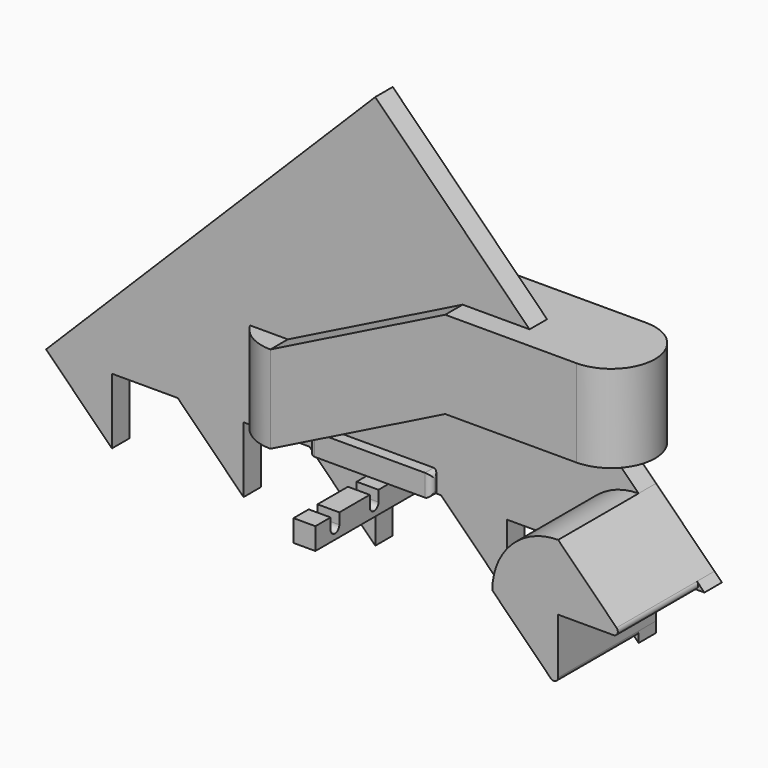
from build123d import *

# Parameters (mm, degrees)
F0_W          = 101.6
F0_H          = 50.8
F0_W_2        = 50.8
F0_H_2        = 101.6
F1_DEPTH      = 50.8
F2_ANGLE_BACK = 90
F2_ANGLE      = 180
F3_DEPTH      = 2.286
F0_W_3        = 43.6525400519
F4_ANGLE_BACK = 90
F4_ANGLE      = 180
F5_W          = 22.098
F5_H          = 6.35
F6_DEPTH      = 25.4
F7_W          = 57.8641055384
F7_H          = 12.7
F7_W_2        = 12.7
F7_H_2        = 49.9071290871
F8_DEPTH      = 25.4
F9_R          = 6.34999
F11_DEPTH     = 25.4
F12_DEPTH     = 142.24
F13_R         = 5.08


# Not quite as in the source:
# - a fillet or chamfer is up to 0.001 mm smaller than in the source, because OpenCascade refuses the exact size


with BuildPart() as f1:
    # F0 (on Front) → F1 (new body, symmetric)
    with BuildSketch(Plane.XZ):
        Polygon((101.6, 203.2), (0, 152.4), (101.6, 152.4), align=None)
        with Locations((50.8, 127)):
            Rectangle(F0_W, F0_H)
        Polygon((0, 152.4), (-101.6, 101.6), (0, 101.6), align=None)
        with Locations((-50.8, 76.2)):
            Rectangle(F0_W, F0_H)
        Polygon((0, 101.6), (0, 50.8), (101.6, 101.6), align=None)
        Polygon((-101.6, 50.8), (-101.6, 0), (0, 50.8), align=None)
        Polygon((101.6, 152.4), (101.6, 101.6), (152.4, 101.6), (152.4, 203.2), (101.6, 203.2), align=None)
        with Locations((177.8, 152.4)):
            Rectangle(F0_W_2, F0_H_2)
        with Locations((228.6, 152.4)):
            Rectangle(F0_W_2, F0_H_2)
    extrude(amount=F1_DEPTH, both=True)

    # F0 (on Front) → F2 (revolve)
    with BuildSketch(Plane.XZ, mode=Mode.PRIVATE) as f2_sk:
        with Locations((279.4, 152.4)):
            Rectangle(F0_W_2, F0_H_2)
    revolve(f2_sk.sketch.rotate(Axis((254, 0, 152.4), (0, 0, -1)), -F2_ANGLE_BACK), axis=Axis((254, 0, 152.4), (0, 0, -1)), revolution_arc=F2_ANGLE)

    # F0 (on Front) → F4 (revolve)
    with BuildSketch(Plane.XZ, mode=Mode.PRIVATE) as f4_sk:
        with Locations((-130.573729974, 50.8)):
            Rectangle(F0_W_3, F0_H_2)
        Polygon((-108.7474599481, 0), (-101.6, 0), (-101.6, 50.8), (-101.6, 101.6), (-108.7474599481, 101.6), align=None)
    revolve(f4_sk.sketch.rotate(Axis((-101.6, 0, 50.8), (0, 0, -1)), -F4_ANGLE_BACK), axis=Axis((-101.6, 0, 50.8), (0, 0, -1)), revolution_arc=F4_ANGLE)


with BuildPart() as f3:
    # F0 (on Front) → F3 (new body)
    with BuildSketch(Plane.XZ):
        Polygon((-108.7474599481, 0), (-101.6, 0), (-101.6, 50.8), (-101.6, 101.6), (-108.7474599481, 101.6), align=None)
    extrude(amount=F3_DEPTH)

    # F10 (on Front) → F11 (join)
    with BuildSketch(Plane.XZ):
        Polygon((-344.3030196818, 38.2558910758), (-382.5589107575, 0), (-306.047128606, 0), align=None)
        Polygon((-306.047128606, 0), (-382.5589107575, 0), (-306.047128606, -76.5117821515), align=None)
        Polygon((-344.3030196818, 38.2558910758), (-306.047128606, 0), (-229.5353464545, 0), (-306.047128606, 76.5117821515), align=None)
        with BuildLine():
            ThreePointArc((-229.5353464545, 0), (-251.945128606, 54.102), (-306.047128606, 76.5117821515))
            Line((-306.047128606, 76.5117821515), (-229.5353464545, 0))
        make_face()
        with BuildLine():
            Line((-267.7912375303, 114.7676732273), (-306.047128606, 76.5117821515))
            ThreePointArc((-306.047128606, 76.5117821515), (-251.945128606, 54.102), (-229.5353464545, 0))
            ThreePointArc((-229.5353464545, 0), (-223.7112338288, 29.2797914101), (-207.125564303, 54.102))
            Line((-207.125564303, 54.102), (-267.7912375303, 114.7676732273))
        make_face()
        with BuildLine():
            ThreePointArc((-207.125564303, 54.102), (-223.7112338288, 29.2797914101), (-229.5353464545, 0))
            Line((-229.5353464545, 0), (-153.023564303, 0))
            Line((-153.023564303, 0), (-207.125564303, 54.102))
        make_face()
        Polygon((-153.023564303, 0), (-229.5353464545, 0), (-153.023564303, -76.5117821515), align=None)
        with BuildLine():
            Line((-229.5353464545, 153.023564303), (-267.7912375303, 114.7676732273))
            Line((-267.7912375303, 114.7676732273), (-207.125564303, 54.102))
            ThreePointArc((-207.125564303, 54.102), (-182.3033557131, 70.6876695257), (-153.023564303, 76.5117821515))
            Line((-153.023564303, 76.5117821515), (-229.5353464545, 153.023564303))
        make_face()
        with BuildLine():
            Line((-207.125564303, 54.102), (-153.023564303, 0))
            Line((-153.023564303, 0), (-76.5117821515, 0))
            Line((-76.5117821515, 0), (-153.023564303, 76.5117821515))
            ThreePointArc((-153.023564303, 76.5117821515), (-182.3033557131, 70.6876695257), (-207.125564303, 54.102))
        make_face()
        with BuildLine():
            Line((-191.2794553788, 191.2794553788), (-229.5353464545, 153.023564303))
            Line((-229.5353464545, 153.023564303), (-153.023564303, 76.5117821515))
            ThreePointArc((-153.023564303, 76.5117821515), (-98.921564303, 54.102), (-76.5117821515, 0))
            ThreePointArc((-76.5117821515, 0), (-70.6876695257, 29.2797914101), (-54.102, 54.102))
            Line((-54.102, 54.102), (-191.2794553788, 191.2794553788))
        make_face()
        Polygon((-38.2558910758, 38.2558910758), (-76.5117821515, 0), (0, 0), align=None)
        Polygon((0, 0), (-76.5117821515, 0), (0, -76.5117821515), align=None)
        with BuildLine():
            ThreePointArc((-54.102, 54.102), (-70.6876695257, 29.2797914101), (-76.5117821515, 0))
            Line((-76.5117821515, 0), (-38.2558910758, 38.2558910758))
            Line((-38.2558910758, 38.2558910758), (-54.102, 54.102))
        make_face()
        with BuildLine():
            Line((-153.023564303, 76.5117821515), (-76.5117821515, 0))
            ThreePointArc((-76.5117821515, 0), (-98.921564303, 54.102), (-153.023564303, 76.5117821515))
        make_face()
        with BuildLine():
            Line((-153.023564303, 229.5353464545), (-191.2794553788, 191.2794553788))
            Line((-191.2794553788, 191.2794553788), (-54.102, 54.102))
            ThreePointArc((-54.102, 54.102), (-29.2797914101, 70.6876695257), (0, 76.5117821515))
            Line((0, 76.5117821515), (-153.023564303, 229.5353464545))
        make_face()
        Polygon((-38.2558910758, 38.2558910758), (0, 0), (76.5117821515, 0), (0, 76.5117821515), align=None)
        with BuildLine():
            Line((-54.102, 54.102), (-38.2558910758, 38.2558910758))
            Line((-38.2558910758, 38.2558910758), (0, 76.5117821515))
            ThreePointArc((0, 76.5117821515), (-29.2797914101, 70.6876695257), (-54.102, 54.102))
        make_face()
        Polygon((-114.7676732273, 267.7912375303), (-153.023564303, 229.5353464545), (0, 76.5117821515), (38.2558910758, 114.7676732273), align=None)
        Polygon((114.7676732273, 38.2558910758), (76.5117821515, 0), (153.023564303, 0), align=None)
        Polygon((153.023564303, 0), (76.5117821515, 0), (153.023564303, -76.5117821515), align=None)
        with BuildLine():
            ThreePointArc((98.921564303, 54.102), (82.3358947773, 29.2797914101), (76.5117821515, 0))
            Line((76.5117821515, 0), (114.7676732273, 38.2558910758))
            Line((114.7676732273, 38.2558910758), (98.921564303, 54.102))
        make_face()
        with BuildLine():
            ThreePointArc((0, 76.5117821515), (54.102, 54.102), (76.5117821515, 0))
            ThreePointArc((76.5117821515, 0), (82.3358947773, 29.2797914101), (98.921564303, 54.102))
            Line((98.921564303, 54.102), (38.2558910758, 114.7676732273))
            Line((38.2558910758, 114.7676732273), (0, 76.5117821515))
        make_face()
        with BuildLine():
            Line((0, 76.5117821515), (76.5117821515, 0))
            ThreePointArc((76.5117821515, 0), (54.102, 54.102), (0, 76.5117821515))
        make_face()
        Polygon((-76.5117821515, 306.047128606), (-114.7676732273, 267.7912375303), (38.2558910758, 114.7676732273), (76.5117821515, 153.023564303), align=None)
        Polygon((114.7676732273, 38.2558910758), (153.023564303, 0), (229.5353464545, 0), (153.023564303, 76.5117821515), align=None)
        with BuildLine():
            Line((98.921564303, 54.102), (114.7676732273, 38.2558910758))
            Line((114.7676732273, 38.2558910758), (153.023564303, 76.5117821515))
            ThreePointArc((153.023564303, 76.5117821515), (123.7437728929, 70.6876695257), (98.921564303, 54.102))
        make_face()
        with BuildLine():
            Line((38.2558910758, 114.7676732273), (98.921564303, 54.102))
            ThreePointArc((98.921564303, 54.102), (123.7437728929, 70.6876695257), (153.023564303, 76.5117821515))
            Line((153.023564303, 76.5117821515), (76.5117821515, 153.023564303))
            Line((76.5117821515, 153.023564303), (38.2558910758, 114.7676732273))
        make_face()
        Polygon((-38.2558910758, 344.3030196818), (-76.5117821515, 306.047128606), (76.5117821515, 153.023564303), (114.7676732273, 191.2794553788), align=None)
        with BuildLine():
            ThreePointArc((251.945128606, 54.102), (235.3594590803, 29.2797914101), (229.5353464545, 0))
            Line((229.5353464545, 0), (306.047128606, 0))
            Line((306.047128606, 0), (251.945128606, 54.102))
        make_face()
        Polygon((306.047128606, 0), (229.5353464545, 0), (306.047128606, -76.5117821515), align=None)
        with BuildLine():
            ThreePointArc((153.023564303, 76.5117821515), (207.125564303, 54.102), (229.5353464545, 0))
            ThreePointArc((229.5353464545, 0), (235.3594590803, 29.2797914101), (251.945128606, 54.102))
            Line((251.945128606, 54.102), (191.2794553788, 114.7676732273))
            Line((191.2794553788, 114.7676732273), (153.023564303, 76.5117821515))
        make_face()
        with BuildLine():
            Line((153.023564303, 76.5117821515), (229.5353464545, 0))
            ThreePointArc((229.5353464545, 0), (207.125564303, 54.102), (153.023564303, 76.5117821515))
        make_face()
        Polygon((153.023564303, 153.023564303), (153.023564303, 76.5117821515), (191.2794553788, 114.7676732273), align=None)
        Polygon((76.5117821515, 153.023564303), (153.023564303, 76.5117821515), (153.023564303, 153.023564303), align=None)
        Polygon((114.7676732273, 191.2794553788), (76.5117821515, 153.023564303), (153.023564303, 153.023564303), align=None)
        Polygon((0, 382.5589107575), (-38.2558910758, 344.3030196818), (114.7676732273, 191.2794553788), (153.023564303, 229.5353464545), align=None)
        with BuildLine():
            Line((251.945128606, 54.102), (306.047128606, 0))
            Line((306.047128606, 0), (382.5589107575, 0))
            Line((382.5589107575, 0), (306.047128606, 76.5117821515))
            ThreePointArc((306.047128606, 76.5117821515), (276.7673371959, 70.6876695257), (251.945128606, 54.102))
        make_face()
        with BuildLine():
            Line((191.2794553788, 114.7676732273), (251.945128606, 54.102))
            ThreePointArc((251.945128606, 54.102), (276.7673371959, 70.6876695257), (306.047128606, 76.5117821515))
            Line((306.047128606, 76.5117821515), (229.5353464545, 153.023564303))
            Line((229.5353464545, 153.023564303), (191.2794553788, 114.7676732273))
        make_face()
        Polygon((153.023564303, 153.023564303), (191.2794553788, 114.7676732273), (229.5353464545, 153.023564303), align=None)
        Polygon((114.7676732273, 191.2794553788), (153.023564303, 153.023564303), (153.023564303, 229.5353464545), align=None)
        Polygon((153.023564303, 229.5353464545), (153.023564303, 153.023564303), (229.5353464545, 153.023564303), align=None)
    extrude(amount=F11_DEPTH)


with BuildPart() as f6:
    # F5 (on Right) → F6 (new body)
    with BuildSketch(Plane.YZ):
        with Locations((-133.0807154845, -3.175)):
            Rectangle(F5_W, F5_H)
        with Locations((129.3012845155, -3.175)):
            Rectangle(F5_W, F5_H)
        with Locations((-76.1847154845, -3.175)):
            Rectangle(F5_W, F5_H)
        with Locations((-41.3867154845, -3.175)):
            Rectangle(F5_W, F5_H)
        with Locations((-19.2887154845, -3.175)):
            Rectangle(F5_W, F5_H)
        with Locations((15.5092845155, -3.175)):
            Rectangle(F5_W, F5_H)
        with Locations((37.6072845155, -3.175)):
            Rectangle(F5_W, F5_H)
        with Locations((72.4052845155, -3.175)):
            Rectangle(F5_W, F5_H)
        with Locations((94.5032845155, -3.175)):
            Rectangle(F5_W, F5_H)
        with BuildLine():
            Line((-122.0317154845, -12.7), (-144.1297154845, -12.7))
            Line((-144.1297154845, -12.7), (-144.1297154845, -25.4))
            Line((-144.1297154845, -25.4), (-115.6817154845, -25.4))
            Line((-115.6817154845, -25.4), (-115.6817154845, -19.05))
            ThreePointArc((-115.6817154845, -19.05), (-120.171843545, -17.1901280605), (-122.0317154845, -12.7))
        make_face()
        with BuildLine():
            Line((111.9022845155, -19.05), (111.9022845155, -25.4))
            Line((111.9022845155, -25.4), (140.3502845155, -25.4))
            Line((140.3502845155, -25.4), (140.3502845155, -12.7))
            Line((140.3502845155, -12.7), (118.2522845155, -12.7))
            ThreePointArc((118.2522845155, -12.7), (116.3924125761, -17.1901280605), (111.9022845155, -19.05))
        make_face()
        with Locations((-133.0807154845, -9.525)):
            Rectangle(F5_W, F5_H)
        with BuildLine():
            Line((-87.2337154845, -12.7), (-109.3317154845, -12.7))
            ThreePointArc((-109.3317154845, -12.7), (-111.1915874239, -17.1901280605), (-115.6817154845, -19.05))
            Line((-115.6817154845, -19.05), (-115.6817154845, -25.4))
            Line((-115.6817154845, -25.4), (-87.2337154845, -25.4))
            Line((-87.2337154845, -25.4), (-87.2337154845, -12.7))
        make_face()
        with BuildLine():
            Line((-65.1357154845, -12.7), (-87.2337154845, -12.7))
            Line((-87.2337154845, -12.7), (-87.2337154845, -25.4))
            Line((-87.2337154845, -25.4), (-58.7857154845, -25.4))
            Line((-58.7857154845, -25.4), (-58.7857154845, -19.05))
            ThreePointArc((-58.7857154845, -19.05), (-63.275843545, -17.1901280605), (-65.1357154845, -12.7))
        make_face()
        with BuildLine():
            Line((-58.7857154845, -19.05), (-58.7857154845, -25.4))
            Line((-58.7857154845, -25.4), (-30.3377154845, -25.4))
            Line((-30.3377154845, -25.4), (-30.3377154845, -12.7))
            Line((-30.3377154845, -12.7), (-52.4357154845, -12.7))
            ThreePointArc((-52.4357154845, -12.7), (-54.2955874239, -17.1901280605), (-58.7857154845, -19.05))
        make_face()
        with BuildLine():
            Line((-30.3377154845, -12.7), (-30.3377154845, -25.4))
            Line((-30.3377154845, -25.4), (-1.8897154845, -25.4))
            Line((-1.8897154845, -25.4), (-1.8897154845, -19.05))
            ThreePointArc((-1.8897154845, -19.05), (-6.379843545, -17.1901280605), (-8.2397154845, -12.7))
            Line((-8.2397154845, -12.7), (-30.3377154845, -12.7))
        make_face()
        with BuildLine():
            Line((-1.8897154845, -19.05), (-1.8897154845, -25.4))
            Line((-1.8897154845, -25.4), (26.5582845155, -25.4))
            Line((26.5582845155, -25.4), (26.5582845155, -12.7))
            Line((26.5582845155, -12.7), (4.4602845155, -12.7))
            ThreePointArc((4.4602845155, -12.7), (2.6004125761, -17.1901280605), (-1.8897154845, -19.05))
        make_face()
        with BuildLine():
            Line((26.5582845155, -12.7), (26.5582845155, -25.4))
            Line((26.5582845155, -25.4), (55.0062845155, -25.4))
            Line((55.0062845155, -25.4), (55.0062845155, -19.05))
            ThreePointArc((55.0062845155, -19.05), (50.516156455, -17.1901280605), (48.6562845155, -12.7))
            Line((48.6562845155, -12.7), (26.5582845155, -12.7))
        make_face()
        with BuildLine():
            Line((55.0062845155, -19.05), (55.0062845155, -25.4))
            Line((55.0062845155, -25.4), (83.4542845155, -25.4))
            Line((83.4542845155, -25.4), (83.4542845155, -12.7))
            Line((83.4542845155, -12.7), (61.3562845155, -12.7))
            ThreePointArc((61.3562845155, -12.7), (59.4964125761, -17.1901280605), (55.0062845155, -19.05))
        make_face()
        with BuildLine():
            Line((83.4542845155, -12.7), (83.4542845155, -25.4))
            Line((83.4542845155, -25.4), (111.9022845155, -25.4))
            Line((111.9022845155, -25.4), (111.9022845155, -19.05))
            ThreePointArc((111.9022845155, -19.05), (107.412156455, -17.1901280605), (105.5522845155, -12.7))
            Line((105.5522845155, -12.7), (83.4542845155, -12.7))
        make_face()
        with Locations((-98.2827154845, -9.525)):
            Rectangle(F5_W, F5_H)
        with Locations((-98.2827154845, -3.175)):
            Rectangle(F5_W, F5_H)
        with Locations((-76.1847154845, -9.525)):
            Rectangle(F5_W, F5_H)
        with Locations((-41.3867154845, -9.525)):
            Rectangle(F5_W, F5_H)
        with Locations((-19.2887154845, -9.525)):
            Rectangle(F5_W, F5_H)
        with Locations((15.5092845155, -9.525)):
            Rectangle(F5_W, F5_H)
        with Locations((37.6072845155, -9.525)):
            Rectangle(F5_W, F5_H)
        with Locations((72.4052845155, -9.525)):
            Rectangle(F5_W, F5_H)
        with Locations((94.5032845155, -9.525)):
            Rectangle(F5_W, F5_H)
        with Locations((129.3012845155, -9.525)):
            Rectangle(F5_W, F5_H)
    extrude(amount=F6_DEPTH)


with BuildPart() as f8:
    # F7 (on Top) → F8 (new body)
    with BuildSketch(Plane.XY):
        Polygon((-9.0009163551, -25.4342753371), (-66.8671883946, -25.4342753371), (-66.8677397098, -38.1342753371), (-9.0009163551, -38.1342753371), align=None)
        with Locations((45.3311364141, -31.7842753371)):
            Rectangle(F7_W, F7_H)
        Polygon((3.6990836449, 37.1728537501), (-66.8650218935, 37.1728537501), (-66.8650218935, 24.4728537501), (-9.0009163551, 24.4728537501), (3.6990836449, 24.4728537501), align=None)
        Polygon((74.2631891833, 37.1728537501), (3.6990836449, 37.1728537501), (3.6990836449, 24.4728537501), (16.3990836449, 24.4728537501), (74.2631891833, 24.4728537501), align=None)
        with Locations((10.0490836449, -31.7842753371)):
            Rectangle(F7_W_2, F7_H)
        with Locations((-2.6509163551, -31.7842753371)):
            Rectangle(F7_W_2, F7_H)
        with Locations((-2.6509163551, -0.4807107935)):
            Rectangle(F7_W_2, F7_H_2)
        with Locations((10.0490836449, -0.4807107935)):
            Rectangle(F7_W_2, F7_H_2)
    extrude(amount=F8_DEPTH)

    # F9 (radius 6.35 in the source; OpenCascade refuses exactly that, so slightly less here)
    f9_edges = [f8.edges().sort_by_distance(p)[0] for p in [
        (-66.867188, -25.434275, 12.7),
        (-66.86774, -38.134275, 12.7),
        (-66.867464, -31.784275, 0),
        (-66.867464, -31.784275, 25.4),
        (-66.865022, 37.172854, 12.7),
        (-66.865022, 24.472854, 12.7),
        (-66.865022, 30.822854, 0),
        (-66.865022, 30.822854, 25.4),
        (74.263189, -38.134275, 12.7),
        (74.263189, -25.434275, 12.7),
        (74.263189, -31.784275, 0),
        (74.263189, -31.784275, 25.4),
        (74.263189, 24.472854, 12.7),
        (74.263189, 37.172854, 12.7),
        (74.263189, 30.822854, 0),
        (74.263189, 30.822854, 25.4),
    ]]
    fillet(f9_edges, radius=F9_R)


with BuildPart() as f12:
    # F10 (on Front) → F12 (new body)
    with BuildSketch(Plane.XZ):
        with BuildLine():
            ThreePointArc((251.945128606, 54.102), (235.3594590803, 29.2797914101), (229.5353464545, 0))
            Line((229.5353464545, 0), (306.047128606, 0))
            Line((306.047128606, 0), (251.945128606, 54.102))
        make_face()
        Polygon((306.047128606, 0), (229.5353464545, 0), (306.047128606, -76.5117821515), align=None)
        with BuildLine():
            Line((251.945128606, 54.102), (306.047128606, 0))
            Line((306.047128606, 0), (382.5589107575, 0))
            Line((382.5589107575, 0), (306.047128606, 76.5117821515))
            ThreePointArc((306.047128606, 76.5117821515), (276.7673371959, 70.6876695257), (251.945128606, 54.102))
        make_face()
    extrude(amount=F12_DEPTH)

    # F13
    f13_edges = [f12.edges().sort_by_distance(p)[0] for p in [
        (382.558911, -71.12, 0),
        (306.047129, -71.12, -76.511782),
    ]]
    fillet(f13_edges, radius=F13_R)


solid = Compound([f1.part, f3.part, f6.part, f8.part, f12.part])
